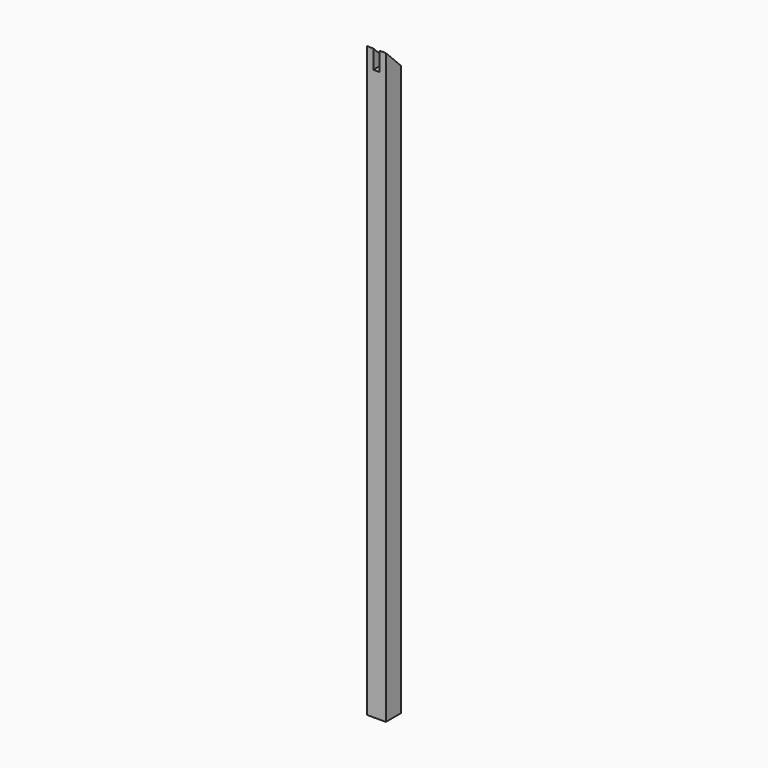
from build123d import *

# Parameters (mm, degrees)
F0_W     = 45
F0_H     = 1407
F1_DEPTH = 22.5
F3_SIZE2 = 44.99999
F3_SIZE  = 44.99999
F2_W     = 15
F2_H     = 45
F4_DEPTH = 45
F5_R     = 9
F6_DEPTH = 30
F9_D     = 3.5
F9_DEPTH = 30
F9_TIP   = 1.0515060833


# Not quite as in the source:
# - a fillet or chamfer is up to 0.001 mm smaller than in the source, because OpenCascade refuses the exact size


with BuildPart() as f1:
    # F0 (on Front) → F1 (new body, symmetric)
    with BuildSketch(Plane.XZ):
        with Locations((0, -490.1653682211)):
            Rectangle(F0_W, F0_H)
    extrude(amount=F1_DEPTH, both=True)

    # F3 (size 45 and 45 in the source; OpenCascade refuses exactly that, so slightly less here)
    f3_edges = [f1.edges().sort_by_distance(p)[0] for p in [
        (0, 22.5, 213.334632),
    ]]
    chamfer(f3_edges, length=F3_SIZE, length2=F3_SIZE2)

    # F2 (on face) → F4 (cut)
    with BuildSketch(Plane.XY.offset(213.3346317789)):
        Rectangle(F2_W, F2_H)
    extrude(amount=-F4_DEPTH, mode=Mode.SUBTRACT)

    # F5 (on face) → F6 (cut)
    with BuildSketch(Plane(origin=(-22.5, 0, 0), x_dir=(0, -1, 0), z_dir=(-1, 0, 0))):
        with Locations((0, 38.3346317789)):
            Circle(F5_R)
        with Locations((0, -311.6653682211)):
            Circle(F5_R)
        with Locations((0, -661.6653682211)):
            Circle(F5_R)
        with Locations((0, -1011.6653682211)):
            Circle(F5_R)
    extrude(amount=-F6_DEPTH, mode=Mode.SUBTRACT)

    # F9
    with Locations(Plane(origin=(0, 22.5, 0), x_dir=(-1, 0, 0), z_dir=(0, 1, 0))):
        with Locations((-10, 103.3346317789), (-10, 63.3346317789), (10, 63.3346317789), (10, 103.3346317789), (10, 143.3346317789), (-10, 143.3346317789)):
            Hole(F9_D / 2, depth=F9_DEPTH)
            with Locations((0, 0, -(F9_DEPTH + F9_TIP / 2))):  # 118° drill point
                Cone(0, F9_D / 2, F9_TIP, mode=Mode.SUBTRACT)


solid = f1.part
